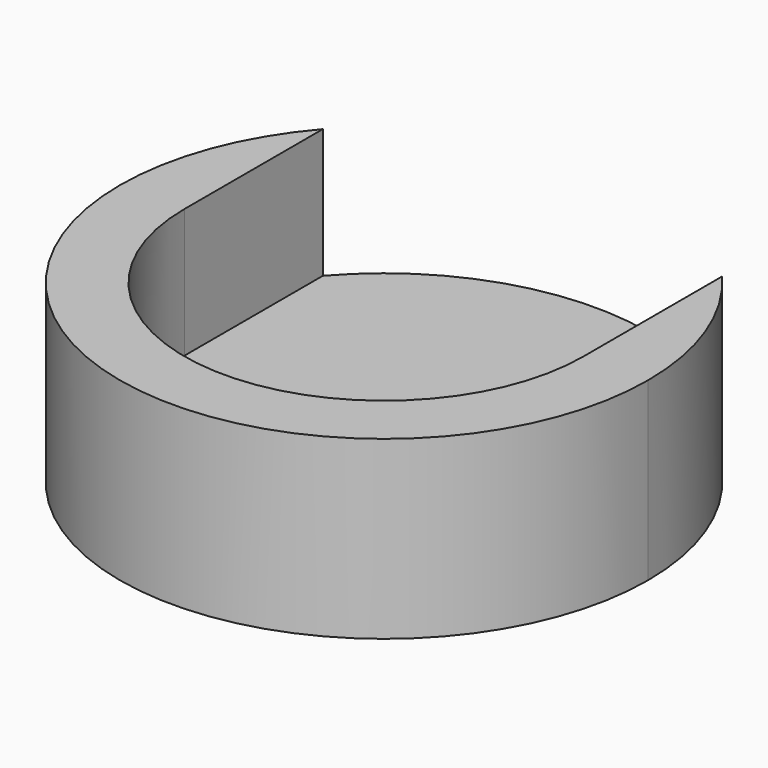
from build123d import *

# Parameters (mm, degrees)
F1_DEPTH = 15
F2_DEPTH = 4


# Not quite as in the source:
# - a feature names something its author has since deleted; it is built from what else it names


with BuildPart() as f1:
    # F0 (on Top) → F1 (new body)
    with BuildSketch(Plane.XY):
        with BuildLine():
            Line((22.5, 0), (17, 0))
            ThreePointArc((17, 0), (0, -17), (-17, 0))
            Line((-17, 0), (-22.5, 0))
            ThreePointArc((-22.5, 0), (0, -22.5), (22.5, 0))
        make_face()
        with BuildLine():
            Line((-22.5, 0), (-17, 0))
            Line((-17, 0), (-17, 14.739402973))
            ThreePointArc((-17, 14.739402973), (-21.0802039838, 7.8660663613), (-22.5, 0))
        make_face()
        with BuildLine():
            Line((17, 14.739402973), (17, 0))
            Line((17, 0), (22.5, 0))
            ThreePointArc((22.5, 0), (21.0802039838, 7.8660663613), (17, 14.739402973))
        make_face()
    extrude(amount=F1_DEPTH)

    # F0 (on Top) → F2 (join)
    with BuildSketch(Plane.XY):
        with BuildLine():
            Line((-17, 0), (17, 0))
            ThreePointArc((17, 0), (0, 17), (-17, 0))
        make_face()
        with BuildLine():
            ThreePointArc((-17, 0), (0, -17), (17, 0))
            Line((17, 0), (-17, 0))
        make_face()
        with BuildLine():
            ThreePointArc((-17, 0), (0, 17), (17, 0))
            Line((17, 0), (17, 14.739402973))
            ThreePointArc((17, 14.739402973), (0, 22.5), (-17, 14.739402973))
            Line((-17, 14.739402973), (-17, 0))
        make_face()
    extrude(amount=F2_DEPTH)


solid = f1.part
